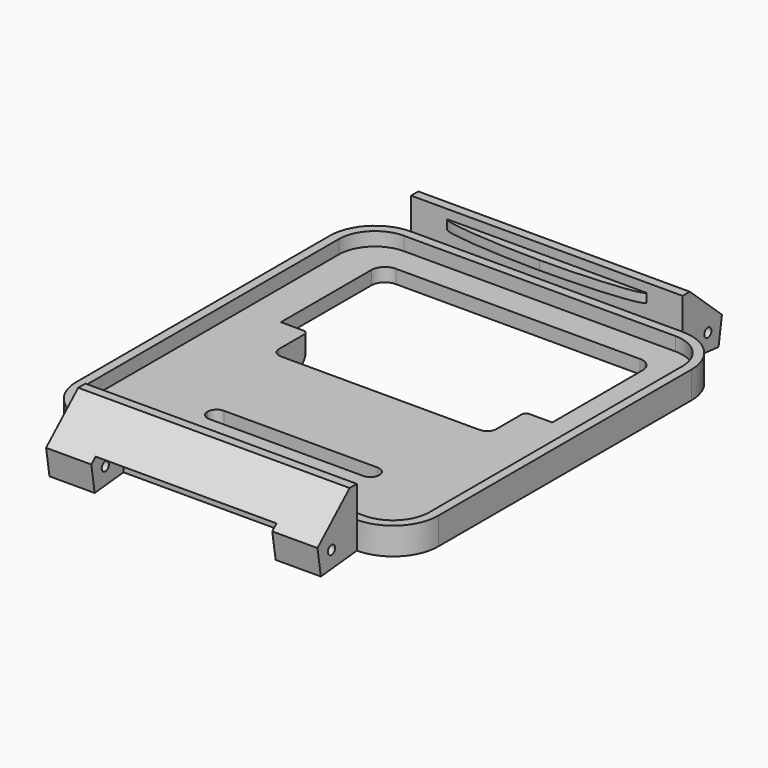
from build123d import *

# Parameters (mm, degrees)
F0_W           = 40
F0_H           = 45
F0_W_2         = 19
F0_H_2         = 2
F0_W_3         = 3
F0_H_3         = 5
F1_DEPTH       = 1.5
F2_DEPTH       = 2.5
F4_DEPTH       = 50
F5_R           = 0.99999
F6_R           = 1.5
F7_R           = 1
F8_R           = 0.5
F9_W           = 40
F9_H           = 45
F9_W_2         = 38
F9_H_2         = 43
F10_DEPTH      = 3
F11_R          = 4
F12_R          = 5
F14_DEPTH      = 15
F14_DEPTH_BACK = 15
F15_W          = 22
F15_H          = 1
F16_DEPTH      = 1
F18_DEPTH      = 1
F19_W          = 22
F19_H          = 1
F20_DEPTH      = 1
F22_DEPTH      = 1
F23_R          = 0.5
F24_DEPTH      = 30
F25_R          = 0.5
F26_DEPTH      = 30
F27_W          = 20
F27_H          = 6
F28_DEPTH      = 3
F28_DEPTH_BACK = 2


# Not quite as in the source:
# - a fillet or chamfer is up to 0.001 mm smaller than in the source, because OpenCascade refuses the exact size


with BuildPart() as f1:
    # F0 (on Top) → F1 (new body)
    with BuildSketch(Plane.XY):
        Rectangle(F0_W, F0_H)
        with Locations((0, -12.5)):
            Rectangle(F0_W_2, F0_H_2, mode=Mode.SUBTRACT)
        Polygon((-15, -0.5), (-15, 4.5), (-15, 18.5), (15, 18.5), (15, 4.5), (15, -0.5), (12, -0.5), (-12, -0.5), align=None, mode=Mode.SUBTRACT)
        with Locations((-13.5, 2)):
            Rectangle(F0_W_3, F0_H_3)
        with Locations((13.5, 2)):
            Rectangle(F0_W_3, F0_H_3)
    extrude(amount=F1_DEPTH)

    # F0 (on Top) → F2 (join)
    with BuildSketch(Plane.XY):
        with Locations((13.5, 2)):
            Rectangle(F0_W_3, F0_H_3)
        with Locations((-13.5, 2)):
            Rectangle(F0_W_3, F0_H_3)
    extrude(amount=-F2_DEPTH)

    # F3 (on face) → F4 (cut)
    with BuildSketch(Plane(origin=(-15, 0, 0), x_dir=(0, -1, 0), z_dir=(-1, 0, 0))):
        with BuildLine():
            add(Edge.make_bspline(
                [(-4.5, 0), (-4.0582373844, -1.0078166901), (-3.0291186922, -2.5), (-2, -2.5)],
                knots=[0, 0, 0, 0, 0.1816780837, 0.1816780837, 0.1816780837, 0.1816780837], degree=3))
            Line((-4.5, 0), (-4.5, -2.5))
            Line((-4.5, -2.5), (-2, -2.5))
        make_face()
        with BuildLine():
            Line((0.5, -2.5), (0.5, 0))
            add(Edge.make_bspline(
                [(-2, -2.5), (-0.9708813078, -2.5), (0.0582373844, -1.0078166901), (0.5, 0)],
                knots=[0.1816780837, 0.1816780837, 0.1816780837, 0.1816780837, 0.3633561673, 0.3633561673, 0.3633561673, 0.3633561673], degree=3))
            Line((-2, -2.5), (0.5, -2.5))
        make_face()
    extrude(amount=-F4_DEPTH, mode=Mode.SUBTRACT)

    # F5 (radius 1 in the source; OpenCascade refuses exactly that, so slightly less here)
    f5_edges = [f1.edges().sort_by_distance(p)[0] for p in [
        (9.5, -11.5, 0.75),
        (9.5, -13.5, 0.75),
        (-9.5, -11.5, 0.75),
        (-9.5, -13.5, 0.75),
    ]]
    fillet(f5_edges, radius=F5_R)

    # F6
    f6_edges = [f1.edges().sort_by_distance(p)[0] for p in [
        (-15, 18.5, 0.75),
        (15, 18.5, 0.75),
    ]]
    fillet(f6_edges, radius=F6_R)

    # F7
    f7_edges = [f1.edges().sort_by_distance(p)[0] for p in [
        (12, -0.5, 0.75),
        (-12, -0.5, 0.75),
    ]]
    fillet(f7_edges, radius=F7_R)

    # F8
    f8_edges = [f1.edges().sort_by_distance(p)[0] for p in [
        (12, 4.5, 0.75),
        (-12, 4.5, 0.75),
    ]]
    fillet(f8_edges, radius=F8_R)

    # F9 (on Top) → F10 (join)
    with BuildSketch(Plane.XY):
        Rectangle(F9_W, F9_H)
        Rectangle(F9_W_2, F9_H_2, mode=Mode.SUBTRACT)
    extrude(amount=F10_DEPTH)

    # F11
    f11_edges = [f1.edges().sort_by_distance(p)[0] for p in [
        (-19, 21.5, 2.25),
        (19, 21.5, 2.25),
        (19, -21.5, 2.25),
        (-19, -21.5, 2.25),
    ]]
    fillet(f11_edges, radius=F11_R)

    # F12
    f12_edges = [f1.edges().sort_by_distance(p)[0] for p in [
        (-20, -22.5, 1.5),
        (20, -22.5, 1.5),
        (20, 22.5, 1.5),
        (-20, 22.5, 1.5),
    ]]
    fillet(f12_edges, radius=F12_R)

    # F13 (on Right) → F14 (join, two sides)
    with BuildSketch(Plane.YZ) as f14_sk:
        Polygon((22.5, 6.5), (22.5, 0), (27.4749371855, -0.5), (27.9395025565, 2.4638115689), (23.5, 6.5), align=None)
        Polygon((-27.4749371855, -0.5), (-22.5, 0), (-22.5, 6.5), (-23.5, 6.5), (-27.9395025565, 2.4638115689), align=None)
    extrude(amount=F14_DEPTH)
    extrude(f14_sk.sketch, amount=-F14_DEPTH_BACK)

    # F15 (on face) → F16 (join)
    with BuildSketch(Plane.XZ.offset(-22.5)):
        with Locations((0, 5)):
            Rectangle(F15_W, F15_H)
    extrude(amount=F16_DEPTH)

    # F17 (on face) → F18 (cut)
    with BuildSketch(Plane.XY.offset(5.5)):
        with BuildLine():
            Line((-11, 21.5), (0, 21.5))
            add(Edge.make_bspline(
                [(0, 21.5), (-5.5, 21.5), (-11, 22), (-11, 22.5)],
                knots=[0, 0, 0, 0, 0.25, 0.25, 0.25, 0.25], degree=3))
            Line((-11, 22.5), (-11, 21.5))
        make_face()
        with BuildLine():
            add(Edge.make_bspline(
                [(11, 22.5), (11, 22), (5.5, 21.5), (0, 21.5)],
                knots=[0.75, 0.75, 0.75, 0.75, 1, 1, 1, 1], degree=3))
            Line((0, 21.5), (11, 21.5))
            Line((11, 21.5), (11, 22.5))
        make_face()
    extrude(amount=-F18_DEPTH, mode=Mode.SUBTRACT)

    # F19 (on face) → F20 (join)
    with BuildSketch(Plane(origin=(0, -22.5, 0), x_dir=(-1, 0, 0), z_dir=(0, 1, 0))):
        with Locations((0, 5)):
            Rectangle(F19_W, F19_H)
    extrude(amount=F20_DEPTH)

    # F21 (on face) → F22 (cut)
    with BuildSketch(Plane.XY.offset(5.5)):
        with BuildLine():
            Line((11, -21.5), (0, -21.5))
            add(Edge.make_bspline(
                [(0, -21.5), (5.5, -21.5), (11, -22), (11, -22.5)],
                knots=[0, 0, 0, 0, 0.25, 0.25, 0.25, 0.25], degree=3))
            Line((11, -22.5), (11, -21.5))
        make_face()
        with BuildLine():
            add(Edge.make_bspline(
                [(-11, -22.5), (-11, -22), (-5.5, -21.5), (0, -21.5)],
                knots=[0.75, 0.75, 0.75, 0.75, 1, 1, 1, 1], degree=3))
            Line((0, -21.5), (-11, -21.5))
            Line((-11, -21.5), (-11, -22.5))
        make_face()
    extrude(amount=-F22_DEPTH, mode=Mode.SUBTRACT)

    # F23 (on face) → F24 (cut)
    with BuildSketch(Plane.YZ.offset(15)):
        with Locations((26, 1.5)):
            Circle(F23_R)
    extrude(amount=-F24_DEPTH, mode=Mode.SUBTRACT)

    # F25 (on face) → F26 (cut)
    with BuildSketch(Plane.YZ.offset(15)):
        with Locations((-26, 1.5)):
            Circle(F25_R)
    extrude(amount=-F26_DEPTH, mode=Mode.SUBTRACT)

    # F27 (on Top) → F28 (cut, two sides)
    with BuildSketch(Plane.XY) as f28_sk:
        with Locations((0, 26.5)):
            Rectangle(F27_W, F27_H)
        with Locations((0, -26.5)):
            Rectangle(F27_W, F27_H)
    extrude(amount=F28_DEPTH, mode=Mode.SUBTRACT)
    extrude(f28_sk.sketch, amount=-F28_DEPTH_BACK, mode=Mode.SUBTRACT)


solid = f1.part
